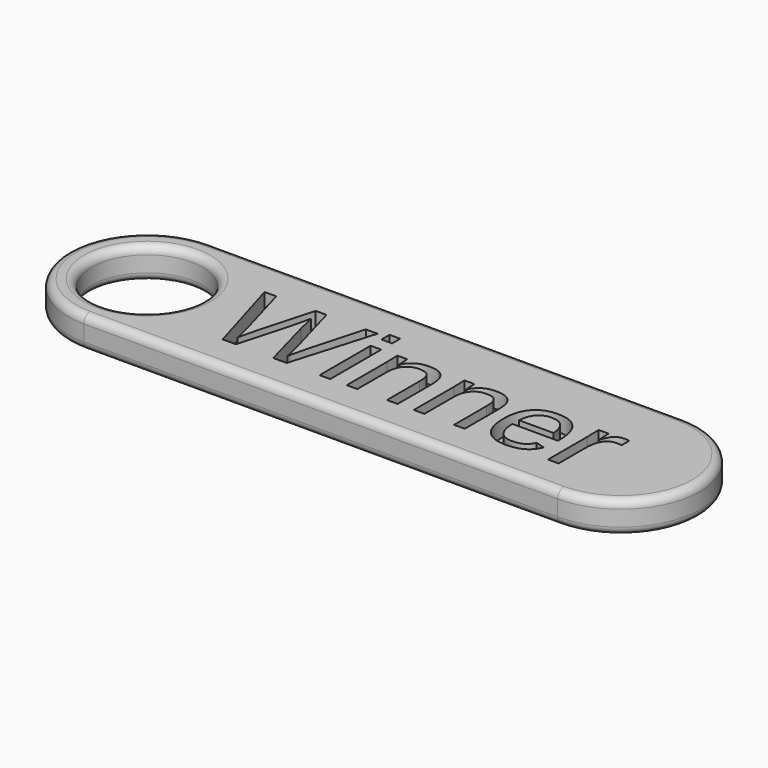
from build123d import *

# Parameters (mm, degrees)
F0_R         = 8.89
F1_DEPTH     = 5.08
F2_TEXT_SIZE = 19.4027777778
F3_DEPTH     = 2.54
F4_R         = 1.27


# Not quite as in the source:
# - Text() gives the source's letters only with a copy of the font that has no kerning and outlines rounded to 1/6400 em; it was checked with that copy


with BuildPart() as f1:
    # F0 (on Top) → F1 (new body)
    with BuildSketch(Plane.XY):
        with BuildLine():
            Line((-38.1, -12.7), (38.1, -12.7))
            ThreePointArc((38.1, -12.7), (50.8, 0), (38.1, 12.7))
            Line((38.1, 12.7), (-38.1, 12.7))
            ThreePointArc((-38.1, 12.7), (-50.8, 0), (-38.1, -12.7))
        make_face()
        with Locations((-38.1, 0)):
            Circle(F0_R, mode=Mode.SUBTRACT)
    extrude(amount=F1_DEPTH)

    # F2 (on face) → F3 (cut)
    with BuildSketch(Plane.XY.offset(5.08)):
        with Locations((-24.3799761285, -6.985)):
            Text('Winner', F2_TEXT_SIZE, font='Arimo', text_align=(TextAlign.LEFT, TextAlign.BOTTOM))
    extrude(amount=-F3_DEPTH, mode=Mode.SUBTRACT)

    # F4
    f4_edges = [f1.edges().sort_by_distance(p)[0] for p in [
        (-50.8, 0, 5.08),
        (0, -12.7, 0),
        (50.8, 0, 0),
        (0, 12.7, 0),
        (-50.8, 0, 0),
        (-46.99, 0, 0),
        (-46.99, 0, 5.08),
    ]]
    fillet(f4_edges, radius=F4_R)


solid = f1.part
